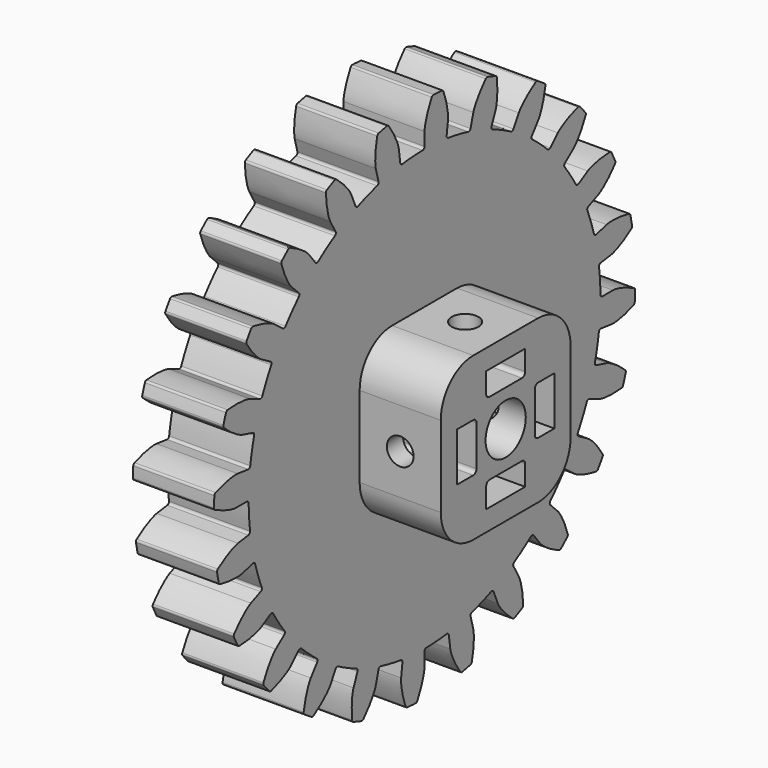
from build123d import *

# Parameters (mm, degrees)
F3_DEPTH        = 10
F3_COPIES_COUNT = 24
F4_R            = 0.3
F6_W            = 20
F6_H            = 20
F7_DEPTH        = 10
F8_R            = 3.1
F9_DEPTH        = 20.0010001
F8_W            = 6
F8_H            = 3
F8_W_2          = 3
F8_H_2          = 6
F10_DEPTH       = 10
F13_D           = 3.3
F13_ON_F11_D    = 3.3
F14_R           = 0.5
F15_R           = 5


# Not quite as in the source:
# - a feature of the source that left no trace in its solid (it failed there, or was rolled back) is left out
# - a pattern or mirror of a feature is missing from the dataset's text; its kind, count and spacing are read off the source's solid
# - a feature names something its author has since deleted; it is built from what else it names


with BuildPart() as f3:
    # F2 (on Right) → F3 (new body)
    with BuildSketch(Plane.YZ):
        with BuildLine():
            ThreePointArc((-27.1075, 0), (0, -27.1075), (27.1075, 0))
            ThreePointArc((27.1075, 0), (1.6886028959, 27.0548549527), (-26.8971242929, 3.3706469737))
            ThreePointArc((-26.8971242929, 3.3706469737), (-27.0548549527, 1.6886028959), (-27.1075, 0))
        make_face()
        with BuildLine():
            ThreePointArc((-27.1075, 0), (-27.0548549527, 1.6886028959), (-26.8971242929, 3.3706469737))
            Line((-26.8971242929, 3.3706469737), (-28.8190213968, 3.6114919275))
            add(Edge.make_bspline(
                [(-32.3745485007, 2.8528248069), (-32.3650622762, 2.8565850615), (-32.1359043919, 2.9471432409), (-31.7059035028, 3.1042803455), (-31.1161219277, 3.2869362209), (-30.5883654103, 3.4218825438), (-30.1257120043, 3.5158329651), (-29.7307254441, 3.5756581186), (-29.4056715724, 3.6084081654), (-29.1515482755, 3.621164149), (-28.9711854201, 3.6213391912), (-28.8614031586, 3.6157734532), (-28.8257780096, 3.6123386409), (-28.8190213968, 3.6114919275)],
                knots=[0.3919177413, 0.3919177413, 0.3919177413, 0.3919177413, 0.3957205093, 0.4838402817, 0.5671932426, 0.6454897173, 0.7183797703, 0.7854288699, 0.8460770668, 0.8995637563, 0.944768275, 0.9797835878, 1, 1, 1, 1], degree=3))
            ThreePointArc((-32.3745485007, 2.8528248069), (-32.4368822636, 2.024516983), (-32.4780271235, 1.1948866739))
            add(Edge.make_bspline(
                [(-32.4780271235, 1.1948866739), (-32.4690820836, 1.1899760495), (-32.2529629859, 1.0716263332), (-31.8458382545, 0.8622408336), (-31.2833459606, 0.6076668868), (-30.7764649783, 0.4081446538), (-30.3290842732, 0.2573953239), (-29.9446020033, 0.1489203689), (-29.6261430697, 0.0760060858), (-29.3755780975, 0.0317504666), (-29.1966367663, 0.0091497973), (-29.0870144378, 0.0010216076), (-29.0512386709, 0), (-29.0444292113, 0)],
                knots=[0.3919177413, 0.3919177413, 0.3919177413, 0.3919177413, 0.3957205093, 0.4838402817, 0.5671932426, 0.6454897173, 0.7183797703, 0.7854288699, 0.8460770668, 0.8995637563, 0.944768275, 0.9797835878, 1, 1, 1, 1], degree=3))
            Line((-29.0444292113, 0), (-27.1075, 0))
        make_face()
    extrude(amount=F3_DEPTH)

    # F3_copies: F3 ×24 about axis
    f3_copies_axis = Axis((0, 0, 0), (1, 0, 0))


with BuildPart() as f3_1:
    add(f3.part)
    for i in range(1, F3_COPIES_COUNT):
        add(f3.part.rotate(f3_copies_axis, i * 360 / F3_COPIES_COUNT))

    # F4
    f4_edges = [f3_1.edges().sort_by_distance(p)[0] for p in [
        (5, -26.897124, 3.370647),
        (5, -32.374549, 2.852825),
        (5, -32.478027, 1.194887),
        (5, -27.1075, 0),
        (5, -26.853015, -3.705693),
        (5, 10.529496, -24.978916),
        (5, 7.015937, -26.183834),
        (5, 3.705693, -26.853015),
        (5, 0, -27.1075),
        (5, -3.370647, -26.897124),
        (5, -7.015937, -26.183834),
        (5, -10.217283, -25.108239),
        (5, -13.55375, -23.475784),
        (5, -16.367628, -21.608269),
        (5, -19.167897, -19.167897),
        (5, -21.402546, -16.635732),
        (5, -23.475784, -13.55375),
        (5, -24.978916, -10.529496),
        (5, -26.183834, -7.015937),
        (5, -26.183834, 7.015937),
        (5, -25.108239, 10.217283),
        (5, -23.475784, 13.55375),
        (5, -21.608269, 16.367628),
        (5, -19.167897, 19.167897),
        (5, -16.635732, 21.402546),
        (5, -13.55375, 23.475784),
        (5, -10.529496, 24.978916),
        (5, -7.015937, 26.183834),
        (5, -3.705693, 26.853015),
        (5, 0, 27.1075),
        (5, 3.370647, 26.897124),
        (5, 7.015937, 26.183834),
        (5, 10.217283, 25.108239),
        (5, 13.55375, 23.475784),
        (5, 16.367628, 21.608269),
        (5, 19.167897, 19.167897),
        (5, 21.402546, 16.635732),
        (5, 23.475784, 13.55375),
        (5, 24.978916, 10.529496),
        (5, 26.183834, 7.015937),
        (5, 26.853015, 3.705693),
        (5, 27.1075, 0),
        (5, 26.897124, -3.370647),
        (5, 26.183834, -7.015937),
        (5, 25.108239, -10.217283),
        (5, 23.475784, -13.55375),
        (5, 21.608269, -16.367628),
        (5, 19.167897, -19.167897),
        (5, 16.635732, -21.402546),
        (5, 13.55375, -23.475784),
        (5, -32.009778, -5.623533),
        (5, 15.204211, -28.72424),
        (5, 13.716655, -29.463594),
        (5, 7.25176, -31.680625),
        (5, 5.623533, -32.009778),
        (5, -1.194887, -32.478027),
        (5, -2.852825, -32.374549),
        (5, -9.560104, -31.062106),
        (5, -11.134767, -30.533047),
        (5, -17.273816, -27.529353),
        (5, -18.657893, -26.610769),
        (5, -23.810346, -22.120521),
        (5, -24.909515, -20.875011),
        (5, -28.72424, -15.204211),
        (5, -29.463594, -13.716655),
        (5, -31.680625, -7.25176),
        (5, -31.062106, 9.560104),
        (5, -30.533047, 11.134767),
        (5, -27.529353, 17.273816),
        (5, -26.610769, 18.657893),
        (5, -22.120521, 23.810346),
        (5, -20.875011, 24.909515),
        (5, -15.204211, 28.72424),
        (5, -13.716655, 29.463594),
        (5, -7.25176, 31.680625),
        (5, -5.623533, 32.009778),
        (5, 1.194887, 32.478027),
        (5, 2.852825, 32.374549),
        (5, 9.560104, 31.062106),
        (5, 11.134767, 30.533047),
        (5, 17.273816, 27.529353),
        (5, 18.657893, 26.610769),
        (5, 23.810346, 22.120521),
        (5, 24.909515, 20.875011),
        (5, 28.72424, 15.204211),
        (5, 29.463594, 13.716655),
        (5, 31.680625, 7.25176),
        (5, 32.009778, 5.623533),
        (5, 32.478027, -1.194887),
        (5, 32.374549, -2.852825),
        (5, 31.062106, -9.560104),
        (5, 30.533047, -11.134767),
        (5, 27.529353, -17.273816),
        (5, 26.610769, -18.657893),
        (5, 22.120521, -23.810346),
        (5, 20.875011, -24.909515),
    ]]
    fillet(f4_edges, radius=F4_R)

    # F6 (on face) → F7 (join)
    with BuildSketch(Plane.YZ.offset(10)):
        Rectangle(F6_W, F6_H)
    extrude(amount=F7_DEPTH)

    # F8 (on face) → F9 (cut, through all)
    with BuildSketch(Plane.YZ.offset(20)):
        Circle(F8_R)
    extrude(amount=-F9_DEPTH, mode=Mode.SUBTRACT)

    # F8 (on face) → F10 (cut)
    with BuildSketch(Plane.YZ.offset(20)):
        with Locations((0, 6)):
            Rectangle(F8_W, F8_H)
        with Locations((6, 0)):
            Rectangle(F8_W_2, F8_H_2)
        with Locations((-6, 0)):
            Rectangle(F8_W_2, F8_H_2)
        with Locations((0, -6)):
            Rectangle(F8_W, F8_H)
    extrude(amount=-F10_DEPTH, mode=Mode.SUBTRACT)

    # F13 (through all)
    with Locations(Plane.XZ.offset(10)):
        with Locations((15, 0)):
            Hole(F13_D / 2)

    # F13 on F11 (through all)
    with Locations(Plane.XY.offset(10)):
        with Locations((15, 0)):
            Hole(F13_ON_F11_D / 2)

    # F14
    f14_edges = [f3_1.edges().sort_by_distance(p)[0] for p in [
        (15, 3, 4.5),
        (15, -3, 4.5),
        (15, -4.5, -3),
        (15, -4.5, 3),
        (15, -3, -4.5),
        (15, 3, -4.5),
        (15, 4.5, -3),
        (15, 4.5, 3),
    ]]
    fillet(f14_edges, radius=F14_R)

    # F15
    f15_edges = [f3_1.edges().sort_by_distance(p)[0] for p in [
        (15, 10, 10),
        (15, 10, -10),
        (15, -10, -10),
        (15, -10, 10),
    ]]
    fillet(f15_edges, radius=F15_R)


solid = f3_1.part
